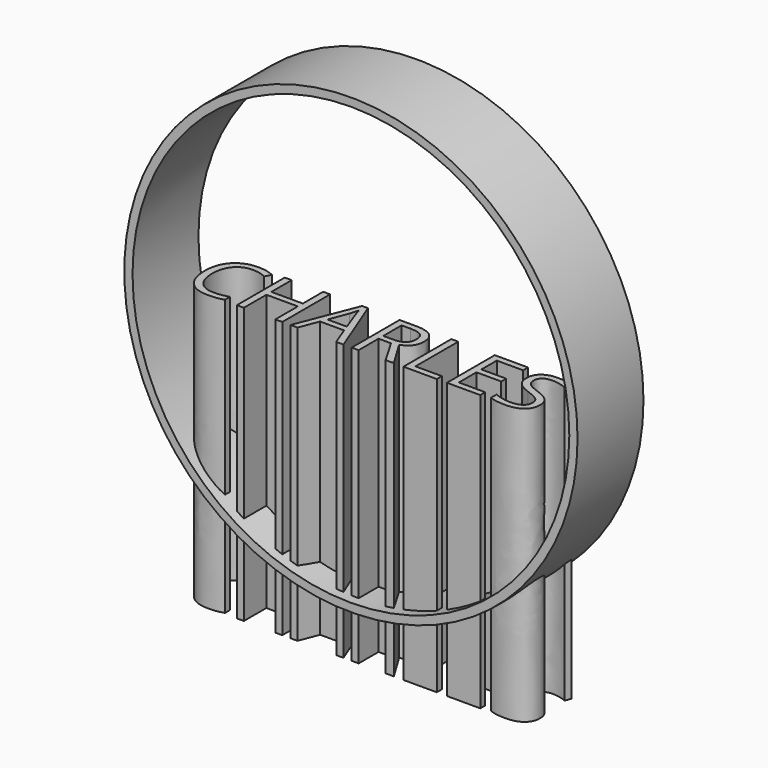
from build123d import *

# Parameters (mm, degrees)
F0_R         = 69.8491538556
F2_DEPTH     = 25.4
F1_R         = 55.9204712171
F3_DEPTH     = 2.54
F4_T         = -2.54
F5_TEXT_SIZE = 25.8125018768
F6_DEPTH     = 85


# Not quite as in the source:
# - Text() gives the source's letters only with a copy of the font that has no kerning and outlines rounded to 1/6400 em; it was checked with that copy


with BuildPart() as f2:
    # F0 (on Front) → F2 (new body)
    with BuildSketch(Plane.XZ):
        Circle(F0_R)
    extrude(amount=F2_DEPTH)

    # F1 (on face) → F3 (join)
    with BuildSketch(Plane.XZ):
        Circle(F1_R)
    extrude(amount=F3_DEPTH)

    # F4
    f4_openings = [f2.faces().sort_by_distance(p)[0] for p in [
        (0, -25.4, 0),
        (0, 0, 0),
    ]]
    offset(amount=F4_T, openings=f4_openings)

    # F5 (on Top) → F6 (join)
    with BuildSketch(Plane.XY):
        with Locations((-56.3850030303, -22.3667919636)):
            Text('CHARLES', F5_TEXT_SIZE, font='Open Sans', text_align=(TextAlign.LEFT, TextAlign.BOTTOM))
    extrude(amount=-F6_DEPTH)


solid = f2.part
